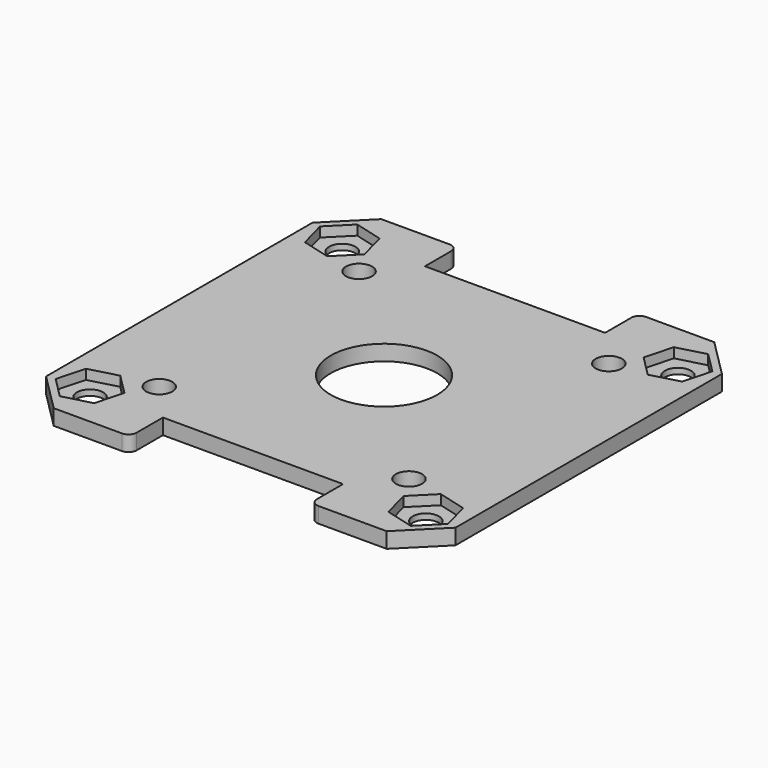
from build123d import *

# Parameters (mm, degrees)
F0_R     = 1.6
F0_R_2   = 6.5
F1_DEPTH = 1.9
F2_R     = 1.6
F3_DEPTH = 1.2


# Not quite as in the source:
# - a feature names something its author has since deleted; it is built from what else it names


with BuildPart() as f1:
    # F0 (on Top) → F1 (new body)
    with BuildSketch(Plane.XY):
        with BuildLine():
            Line((15.7910159975, 25.3955767816), (11.1241112417, 30.0624815375))
            Line((11.1241112417, 30.0624815375), (2.7910159975, 30.0624815375))
            ThreePointArc((2.7910159975, 30.0624815375), (2.0839092163, 29.7695883186), (1.7910159975, 29.0624815375))
            Line((1.7910159975, 29.0624815375), (1.7910159975, 25.0624815375))
            Line((1.7910159975, 25.0624815375), (-20.2089840025, 25.0624815375))
            Line((-20.2089840025, 25.0624815375), (-20.2089840025, 29.0624815375))
            ThreePointArc((-20.2089840025, 29.0624815375), (-20.5018772213, 29.7695883186), (-21.2089840025, 30.0624815375))
            Line((-21.2089840025, 30.0624815375), (-29.5420792466, 30.0624815375))
            Line((-29.5420792466, 30.0624815375), (-34.2089840025, 25.3955767816))
            Line((-34.2089840025, 25.3955767816), (-34.2089840025, -15.2706137067))
            Line((-34.2089840025, -15.2706137067), (-29.5420792466, -19.9375184625))
            Line((-29.5420792466, -19.9375184625), (-21.2089840025, -19.9375184625))
            ThreePointArc((-21.2089840025, -19.9375184625), (-20.5018772213, -19.6446252437), (-20.2089840025, -18.9375184625))
            Line((-20.2089840025, -18.9375184625), (-20.2089840025, -14.9375184625))
            Line((-20.2089840025, -14.9375184625), (1.7910159975, -14.9375184625))
            Line((1.7910159975, -14.9375184625), (1.7910159975, -18.9375184625))
            ThreePointArc((1.7910159975, -18.9375184625), (2.0839092163, -19.6446252437), (2.7910159975, -19.9375184625))
            Line((2.7910159975, -19.9375184625), (11.1241112417, -19.9375184625))
            Line((11.1241112417, -19.9375184625), (15.7910159975, -15.2706137067))
            Line((15.7910159975, -15.2706137067), (15.7910159975, 25.3955767816))
        make_face()
        with Locations((-29.7089840025, -14.1875184625)):
            Circle(F0_R, mode=Mode.SUBTRACT)
        with Locations((-24.4589840025, -10.1875184625)):
            Circle(F0_R, mode=Mode.SUBTRACT)
        with Locations((11.2910159975, -14.1875184625)):
            Circle(F0_R, mode=Mode.SUBTRACT)
        with Locations((6.0410159975, -10.1875184625)):
            Circle(F0_R, mode=Mode.SUBTRACT)
        with Locations((-24.4589840025, 20.3124815375)):
            Circle(F0_R, mode=Mode.SUBTRACT)
        with Locations((-29.7089840025, 24.3124815375)):
            Circle(F0_R, mode=Mode.SUBTRACT)
        with Locations((-9.2089840025, 5.0624815375)):
            Circle(F0_R_2, mode=Mode.SUBTRACT)
        with Locations((6.0410159975, 20.3124815375)):
            Circle(F0_R, mode=Mode.SUBTRACT)
        with Locations((11.2910159975, 24.3124815375)):
            Circle(F0_R, mode=Mode.SUBTRACT)
    extrude(amount=F1_DEPTH)

    # F2 (on face) → F3 (cut)
    with BuildSketch(Plane.XY.offset(1.9)):
        Polygon((-30.6354453237, 27.7700822596), (-33.1665847246, 25.2389428587), (-32.2401234033, 21.7813421366), (-28.7825226812, 20.8548808153), (-26.2513832804, 23.3860202162), (-27.1778446016, 26.8436209383), align=None)
        with Locations((-29.7089840025, 24.3124815375)):
            Circle(F2_R, mode=Mode.SUBTRACT)
        Polygon((14.7486167196, 25.2389428587), (12.2174773188, 27.7700822596), (8.7598765967, 26.8436209383), (7.8334152754, 23.3860202162), (10.3645546763, 20.8548808153), (13.8221553984, 21.7813421366), align=None)
        with Locations((11.2910159975, 24.3124815375)):
            Circle(F2_R, mode=Mode.SUBTRACT)
        Polygon((12.2174773188, -17.6451191847), (14.7486167196, -15.1139797838), (13.8221553984, -11.6563790617), (10.3645546763, -10.7299177404), (7.8334152754, -13.2610571413), (8.7598765967, -16.7186578634), align=None)
        with Locations((11.2910159975, -14.1875184625)):
            Circle(F2_R, mode=Mode.SUBTRACT)
        Polygon((-33.1665847246, -15.1139797838), (-30.6354453237, -17.6451191847), (-27.1778446016, -16.7186578634), (-26.2513832804, -13.2610571413), (-28.7825226812, -10.7299177404), (-32.2401234033, -11.6563790617), align=None)
        with Locations((-29.7089840025, -14.1875184625)):
            Circle(F2_R, mode=Mode.SUBTRACT)
    extrude(amount=-F3_DEPTH, mode=Mode.SUBTRACT)


solid = f1.part
